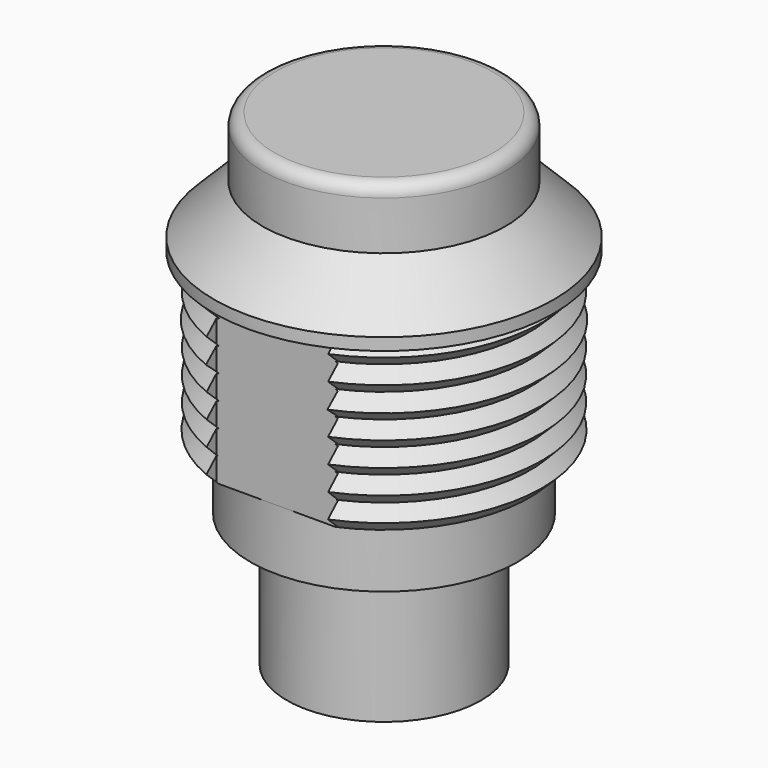
from build123d import *

# Parameters (mm, degrees)
F2_W      = 6
F2_H      = 7
F10_SIZE2 = 1.99999
F10_SIZE  = 1.99999
F11_R     = 0.5
F12_W     = 5
F12_H     = 3.4022161548
F12_H_2   = 4.2761773802
F13_DEPTH = 15


# Not quite as in the source:
# - a fillet or chamfer is up to 0.001 mm smaller than in the source, because OpenCascade refuses the exact size


with BuildPart() as f1:
    # F0 (on Front) → F1 (revolve)
    with BuildSketch(Plane.XZ):
        Polygon((0, 8), (0, 0), (4, 0), (4, 5.5), (5.5, 5.5), (5.5, 8), align=None)
    revolve(axis=Axis((0, 0, 8.8947357469), (0, 0, 1)))

    # F2 (on Front) → F3 (revolve)
    with BuildSketch(Plane.XZ):
        with Locations((3, 11.5)):
            Rectangle(F2_W, F2_H)
    revolve(axis=Axis((0, 0, 12.8918935508), (0, 0, 1)))

    # F6 (on Front) → F7 (revolve)
    with BuildSketch(Plane.XZ):
        Polygon((-6.5108180568, 8.5108180568), (-6, 8), (0, 8), (0, 15), (-5.9985076077, 15), (-6.5, 14.5), (-6, 14), (-6.5, 13.5), (-6, 13), (-6.532786414, 12.5), (-6, 12), (-6.5, 11.5), (-6, 11), (-6.5, 10.5), (-6, 10), (-6.5, 9.5), (-6.0216361135, 9), align=None)
    revolve(axis=Axis((0, 0, 9.6160949171), (0, 0, 1)))

    # F8 (on Front) → F9 (revolve)
    with BuildSketch(Plane.XZ):
        Polygon((-7, 15), (0, 15), (0, 20), (-5, 20), (-5, 17.5), (-7, 17.5), align=None)
    revolve(axis=Axis((0, 0, 18.9704594016), (0, 0, 1)))

    # F10 (size 2 and 2 in the source; OpenCascade refuses exactly that, so slightly less here)
    f10_edges = [f1.edges().sort_by_distance(p)[0] for p in [
        (7, 0, 17.5),
    ]]
    chamfer(f10_edges, length=F10_SIZE, length2=F10_SIZE2)

    # F11
    f11_edges = [f1.edges().sort_by_distance(p)[0] for p in [
        (5, 0, 20),
    ]]
    fillet(f11_edges, radius=F11_R)

    # F12 (on Top) → F13 (cut, through all)
    with BuildSketch(Plane.XY):
        with Locations((0, 7.2011080774)):
            Rectangle(F12_W, F12_H)
        with Locations((0, -7.6380886901)):
            Rectangle(F12_W, F12_H_2)
    extrude(amount=F13_DEPTH, mode=Mode.SUBTRACT)


solid = f1.part
